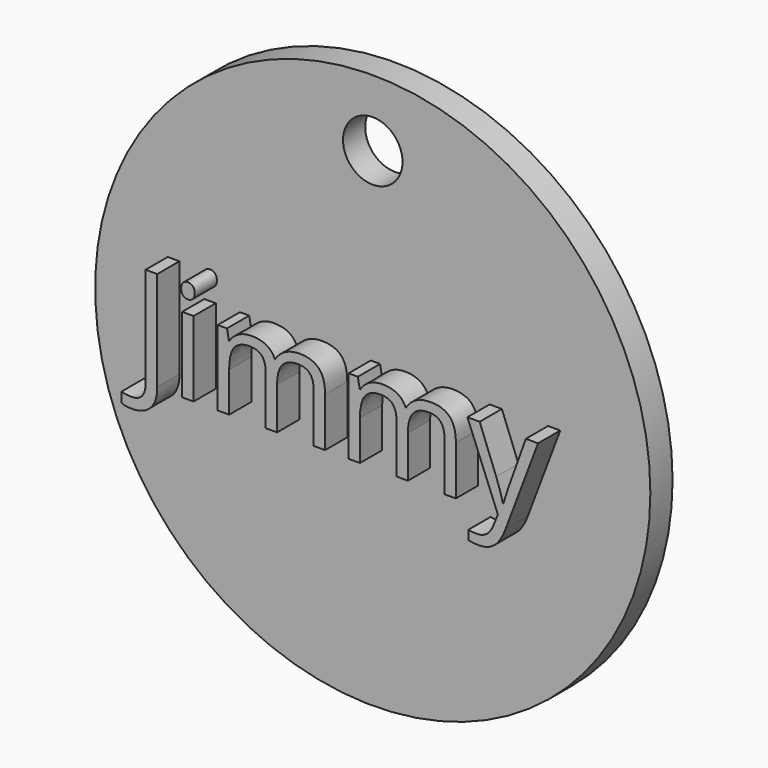
from build123d import *

# Parameters (mm, degrees)
F0_R         = 31.75
F1_DEPTH     = 3.175
F2_TEXT_SIZE = 16.0860415134
F3_DEPTH     = 3.175
F4_R         = 3.402770393
F5_DEPTH     = 12.7


# Not quite as in the source:
# - Text() gives the source's letters only with a copy of the font that has no kerning and outlines rounded to 1/6400 em; it was checked with that copy


with BuildPart() as f1:
    # F0 (on Front) → F1 (new body)
    with BuildSketch(Plane.XZ):
        Circle(F0_R)
    extrude(amount=F1_DEPTH)

    # F2 (on face) → F3 (join)
    with BuildSketch(Plane.XZ.offset(3.175)):
        with Locations((-24.9366499484, -5.6727915071)):
            Text('Jimmy', F2_TEXT_SIZE, font='Open Sans', text_align=(TextAlign.LEFT, TextAlign.BOTTOM))
    extrude(amount=F3_DEPTH)

    # F4 (on face) → F5 (cut, symmetric)
    with BuildSketch(Plane.XZ.offset(3.175)):
        with Locations((0, 24.1093654186)):
            Circle(F4_R)
    extrude(amount=F5_DEPTH, both=True, mode=Mode.SUBTRACT)


solid = f1.part
